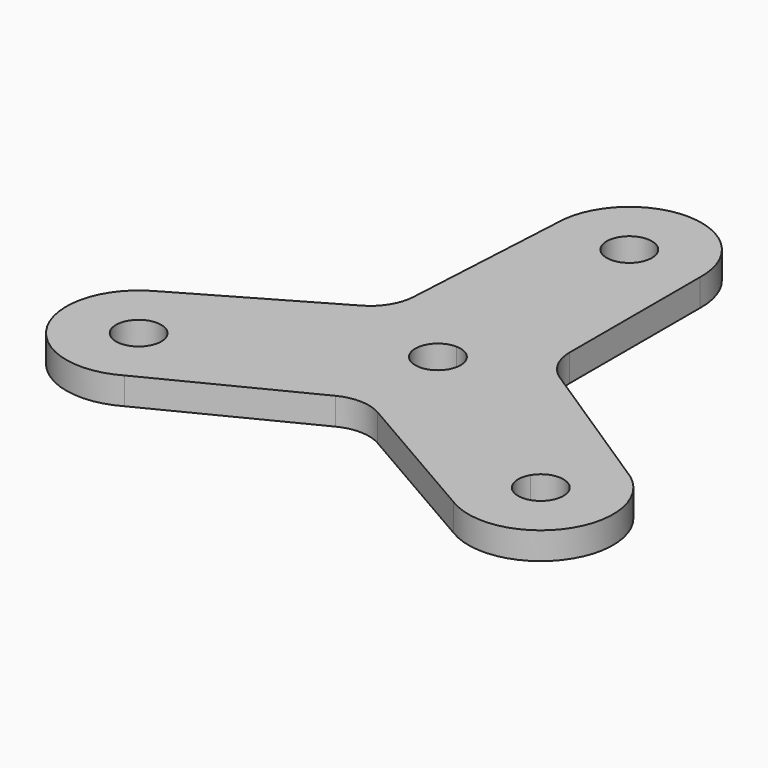
from build123d import *

# Parameters (mm, degrees)
F1_DEPTH = 3


# Not quite as in the source:
# - a feature names something its author has since deleted; it is built from what else it names


with BuildPart() as f1:
    # F0 (on Top) → F1 (new body)
    with BuildSketch(Plane.XY):
        with BuildLine():
            Line((8.3654914828, 7.7478343503), (8.3654914828, 25.7808157751))
            ThreePointArc((8.3654914828, 25.7808157751), (0.4767203504, 33.9966565171), (-7.631576467, 25.9973895632))
            Line((-7.631576467, 25.9973895632), (-8.6528857034, 7.4260866897))
            ThreePointArc((-8.6528857034, 7.4260866897), (-9.3855131516, 5.0826540918), (-11.1453419747, 3.3705145438))
            Line((-11.1453419747, 3.3705145438), (-26.7623619946, -5.6459761686))
            ThreePointArc((-26.7623619946, -5.6459761686), (-29.9331032244, -16.585772745), (-18.951386422, -19.6081302933))
            Line((-18.951386422, -19.6081302933), (-2.3575117339, -11.2069586004))
            ThreePointArc((-2.3575117339, -11.2069586004), (0.038274152, -10.6697162831), (2.400944907, -11.3377029763))
            Line((2.400944907, -11.3377029763), (18.0179649268, -20.3541936886))
            ThreePointArc((18.0179649268, -20.3541936886), (29.0774772891, -17.6302378543), (26.204057304, -6.6086133521))
            Line((26.204057304, -6.6086133521), (10.6314918524, 3.5615178285))
            ThreePointArc((10.6314918524, 3.5615178285), (8.9683334147, 5.3677081091), (8.3654914828, 7.7478343503))
        make_face()
        with BuildLine():
            ThreePointArc((-20.451386422, -12.679927063), (-25.3707248656, -13.3098488797), (-20.7688276181, -11.4607318089))
            ThreePointArc((-20.7688276181, -11.4607318089), (-20.5320479783, -12.0500052463), (-20.451386422, -12.679927063))
        make_face(mode=Mode.SUBTRACT)
        with BuildLine():
            ThreePointArc((24.704057304, -13.5368165824), (21.5399163779, -15.9469860432), (20.0569238399, -12.25626284))
            ThreePointArc((20.0569238399, -12.25626284), (22.8681982302, -11.1266471215), (24.704057304, -13.5368165824))
        make_face(mode=Mode.SUBTRACT)
        with BuildLine():
            ThreePointArc((-7.9164689421, -4.2812988086), (-7.6979940139, 4.6627125327), (0.127531223, 8.9990963873))
            ThreePointArc((0.127531223, 8.9990963873), (6.4088915191, 6.3187110629), (9, 0))
            ThreePointArc((9, 0), (8.6421794957, -2.5125153857), (7.5971703192, -4.8252464332))
            ThreePointArc((7.5971703192, -4.8252464332), (-0.315369081, -8.9944728774), (-7.9164689421, -4.2812988086))
        make_face(mode=Mode.SUBTRACT)
        with BuildLine():
            ThreePointArc((2.868423533, 25.9973895632), (2.1236210505, 24.217141919), (0.3329981933, 23.4976405667))
            ThreePointArc((0.3329981933, 23.4976405667), (-1.3867739845, 27.7776372074), (2.868423533, 25.9973895632))
        make_face(mode=Mode.SUBTRACT)
        with BuildLine():
            ThreePointArc((0.0354253397, 2.4997489965), (1.7802476442, 1.7551975175), (2.5, 0))
            ThreePointArc((2.5, 0), (2.3734655501, -0.7852778377), (2.0066709741, -1.4910639161))
            Line((2.0066709741, -1.4910639161), (7.5971703192, -4.8252464332))
            ThreePointArc((7.5971703192, -4.8252464332), (8.6421794957, -2.5125153857), (9, 0))
            ThreePointArc((9, 0), (6.4088915191, 6.3187110629), (0.127531223, 8.9990963873))
            Line((0.127531223, 8.9990963873), (0.0354253397, 2.4997489965))
        make_face()
        with BuildLine():
            ThreePointArc((-2.239906233, -1.1103243073), (-2.1149683962, 1.333007383), (0.0354253397, 2.4997489965))
            Line((0.0354253397, 2.4997489965), (0.127531223, 8.9990963873))
            ThreePointArc((0.127531223, 8.9990963873), (-7.6979940139, 4.6627125327), (-7.9164689421, -4.2812988086))
            Line((-7.9164689421, -4.2812988086), (-2.239906233, -1.1103243073))
        make_face()
        with BuildLine():
            Line((7.5971703192, -4.8252464332), (2.0066709741, -1.4910639161))
            ThreePointArc((2.0066709741, -1.4910639161), (-0.2232494881, -2.4900119811), (-2.239906233, -1.1103243073))
            Line((-2.239906233, -1.1103243073), (-7.9164689421, -4.2812988086))
            ThreePointArc((-7.9164689421, -4.2812988086), (-0.315369081, -8.9944728774), (7.5971703192, -4.8252464332))
        make_face()
    extrude(amount=F1_DEPTH)


solid = f1.part
